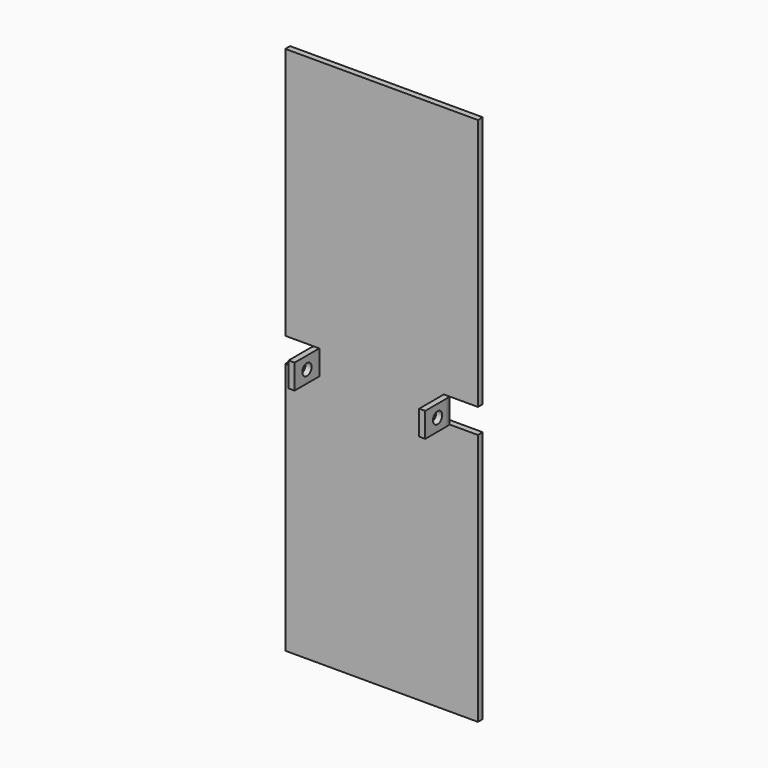
from build123d import *

# Parameters (mm, degrees)
F0_W        = 101.6
F0_H        = 279.4
F1_DEPTH    = 3.175
F2_W        = 3.175
F2_H        = 12.99972
F3_DEPTH    = 16.27124
F2_W_2      = 14.77137
F4_DEPTH    = 25.4
F5_T1_DEPTH = 12.99972
F7_D        = 6.10108


# Not quite as in the source:
# - a fillet or chamfer that OpenCascade refuses, or shapes differently, is made with other operations: its cross-section is extruded or revolved along the edge and cut away or added


with BuildPart() as f1:
    # F0 (on Front) → F1 (new body)
    with BuildSketch(Plane.XZ):
        Rectangle(F0_W, F0_H)
    extrude(amount=F1_DEPTH)

    # F2 (on face) → F3 (join)
    with BuildSketch(Plane.XZ.offset(3.175)):
        with Locations((34.44113, 0)):
            Rectangle(F2_W, F2_H)
        with Locations((-34.44113, 0)):
            Rectangle(F2_W, F2_H)
    extrude(amount=F3_DEPTH)

    # F2 (on face) → F4 (cut)
    with BuildSketch(Plane.XZ.offset(3.175)):
        with Locations((43.414315, 0)):
            Rectangle(F2_W_2, F2_H)
        with Locations((-43.414315, 0)):
            Rectangle(F2_W_2, F2_H)
    extrude(amount=-F4_DEPTH, mode=Mode.SUBTRACT)

    # F5: fillet of radius 5.08 on 2 edges, made by hand

    # F5_s2 → F5_t1 (cut)
    with BuildSketch(Plane.XY.offset(-6.49986)):
        with BuildLine():
            ThreePointArc((30.94863, 0), (34.5407324484, -1.4878975516), (36.02863, -5.08))
            Line((36.02863, -5.08), (36.02863, 0))
            Line((36.02863, 0), (30.94863, 0))
        make_face()
        with BuildLine():
            ThreePointArc((-30.94863, 0), (-34.5407324484, -1.4878975516), (-36.02863, -5.08))
            Line((-36.02863, -5.08), (-36.02863, 0))
            Line((-36.02863, 0), (-30.94863, 0))
        make_face()
    extrude(amount=F5_T1_DEPTH, mode=Mode.SUBTRACT)

    # F7 (through all)
    with Locations(Plane.YZ.offset(36.02863)):
        with Locations((-11.31062, 0)):
            Hole(F7_D / 2)


solid = f1.part
